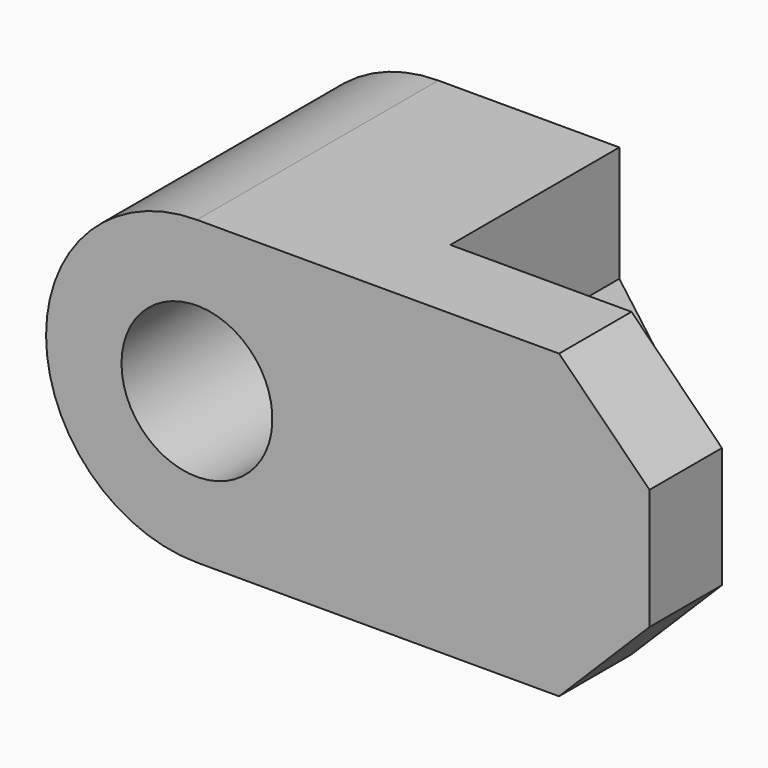
from build123d import *

# Parameters (mm, degrees)
F0_W      = 60
F0_H      = 30
F1_DEPTH  = 30
F2_R      = 14.99999
F4_DEPTH  = 45.974
F5_DEPTH  = 11.5
F7_DEPTH  = 11.5
F8_R      = 7.5
F9_DEPTH  = 31
F11_DEPTH = 25.4
F13_DEPTH = 25.4


# Not quite as in the source:
# - a fillet or chamfer is up to 0.001 mm smaller than in the source, because OpenCascade refuses the exact size


with BuildPart() as f1:
    # F0 (on Front) → F1 (new body)
    with BuildSketch(Plane.XZ):
        with Locations((-1.155378297, 6.3267682405)):
            Rectangle(F0_W, F0_H)
    extrude(amount=F1_DEPTH)

    # F2 (radius 15 in the source; OpenCascade refuses exactly that, so slightly less here)
    f2_edges = [f1.edges().sort_by_distance(p)[0] for p in [
        (-31.155378, -15, 21.326768),
        (-31.155378, -15, -8.673232),
    ]]
    fillet(f2_edges, radius=F2_R)

    # F3 (on face) → F4 (cut)
    with BuildSketch(Plane.XY.offset(21.3267682405)):
        Polygon((28.844621703, 0), (1.844621703, 0), (28.844621703, -21), align=None)
    extrude(amount=-F4_DEPTH, mode=Mode.SUBTRACT)

    # F3 (on face) → F5 (cut)
    with BuildSketch(Plane.XY.offset(21.3267682405)):
        Polygon((28.844621703, -21), (1.844621703, 0), (1.844621703, -21), align=None)
    extrude(amount=-F5_DEPTH, mode=Mode.SUBTRACT)

    # F6 (on face) → F7 (cut)
    with BuildSketch(Plane(origin=(0, 0, -8.6732317595), x_dir=(1, 0, 0), z_dir=(0, 0, -1))):
        Polygon((1.844621703, 21), (1.844621703, 0), (28.844621703, 21), align=None)
    extrude(amount=-F7_DEPTH, mode=Mode.SUBTRACT)

    # F8 (on face) → F9 (cut)
    with BuildSketch(Plane(origin=(0, 0, 0), x_dir=(-1, 0, 0), z_dir=(0, 1, 0))):
        with Locations((16.155378297, 6.3267682405)):
            Circle(F8_R)
    extrude(amount=-F9_DEPTH, mode=Mode.SUBTRACT)

    # F10 (on face) → F11 (cut)
    with BuildSketch(Plane(origin=(0, -21, 0), x_dir=(-1, 0, 0), z_dir=(0, 1, 0))):
        Polygon((-28.844621703, 0.3183682405), (-28.844621703, -8.6732317595), (-19.844621703, -8.6732317595), align=None)
    extrude(amount=-F11_DEPTH, mode=Mode.SUBTRACT)

    # F12 (on face) → F13 (cut)
    with BuildSketch(Plane(origin=(0, -21, 0), x_dir=(-1, 0, 0), z_dir=(0, 1, 0))):
        Polygon((-19.853021703, 21.3267682405), (-28.844621703, 21.3267682405), (-28.844621703, 12.3267682405), align=None)
    extrude(amount=-F13_DEPTH, mode=Mode.SUBTRACT)


solid = f1.part
